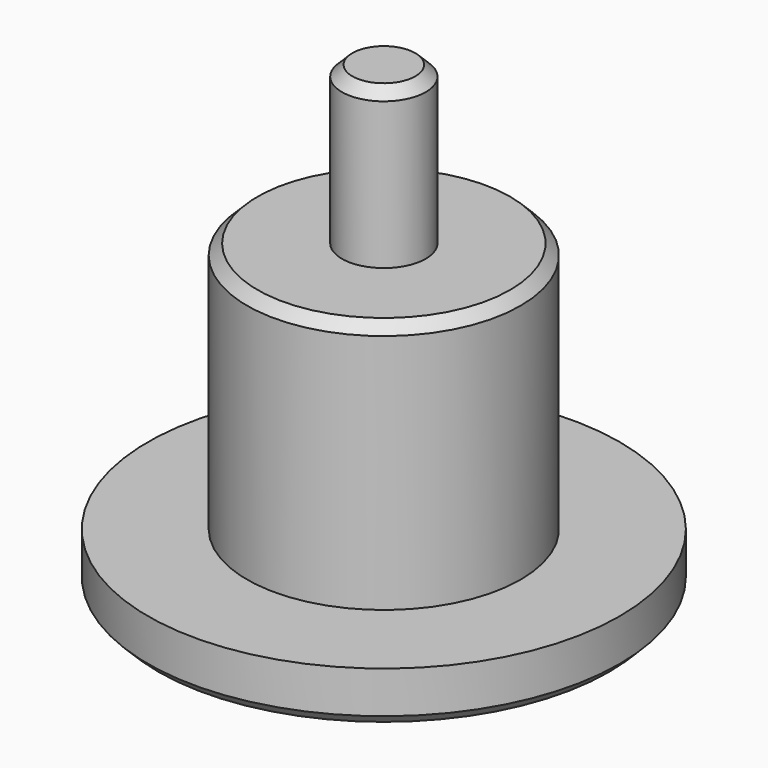
from build123d import *

# Parameters (mm, degrees)
F0_R     = 22.5
F1_DEPTH = 5
F2_R     = 13.05
F3_DEPTH = 29
F4_R     = 4
F5_DEPTH = 44
F6_SIZE  = 1


# Not quite as in the source:
# - a feature names something its author has since deleted; it is built from what else it names


with BuildPart() as f1:
    # F0 (on Top) → F1 (new body)
    with BuildSketch(Plane.XY):
        Circle(F0_R)
    extrude(amount=F1_DEPTH)

    # F2 (on Top) → F3 (join)
    with BuildSketch(Plane.XY):
        Circle(F2_R)
    extrude(amount=F3_DEPTH)

    # F4 (on Top) → F5 (join)
    with BuildSketch(Plane.XY):
        Circle(F4_R)
    extrude(amount=F5_DEPTH)

    # F6
    f6_edges = [f1.edges().sort_by_distance(p)[0] for p in [
        (-22.5, 0, 0),
        (-13.05, 0, 29),
        (-4, 0, 44),
    ]]
    chamfer(f6_edges, length=F6_SIZE)


solid = f1.part
